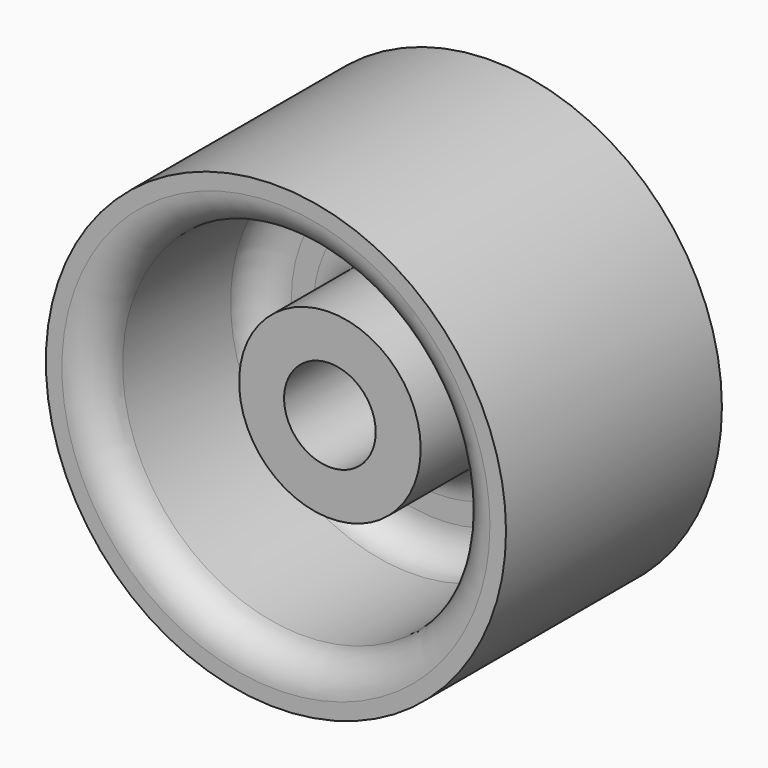
from build123d import *

# Parameters (mm, degrees)
F0_R          = 86.6272823849
F1_DEPTH      = 25.4
F2_R          = 86.6272823849
F2_R_2        = 67.8769245924
F3_DEPTH      = 76.2
F4_R          = 34.1816109176
F4_R_2        = 17.2424518984
F5_DEPTH      = 50.8
F5_DEPTH_BACK = 50.8
F6_R          = 16.8190059926
F7_DEPTH      = 50.8
F8_R          = 12.7
F9_R          = 12.7


with BuildPart() as f1:
    # F0 (on Front) → F1 (new body)
    with BuildSketch(Plane.XZ):
        Circle(F0_R)
    extrude(amount=F1_DEPTH)

    # F2 (on face) → F3 (join)
    with BuildSketch(Plane.XZ.offset(25.4)):
        Circle(F2_R)
        Circle(F2_R_2, mode=Mode.SUBTRACT)
    extrude(amount=F3_DEPTH)

    # F4 (on face) → F5 (join, two sides)
    with BuildSketch(Plane.XZ.offset(25.4)) as f5_sk:
        Circle(F4_R)
        Circle(F4_R_2, mode=Mode.SUBTRACT)
    extrude(amount=F5_DEPTH)
    extrude(f5_sk.sketch, amount=-F5_DEPTH_BACK)

    # F6 (on face) → F7 (cut)
    with BuildSketch(Plane.XZ.offset(25.4)):
        Circle(F6_R)
    extrude(amount=-F7_DEPTH, mode=Mode.SUBTRACT)

    # F8
    f8_edges = [f1.edges().sort_by_distance(p)[0] for p in [
        (-67.876925, -101.6, 0),
    ]]
    fillet(f8_edges, radius=F8_R)

    # F9
    f9_edges = [f1.edges().sort_by_distance(p)[0] for p in [
        (-67.876925, -25.4, 0),
        (-34.181611, -25.4, 0),
    ]]
    fillet(f9_edges, radius=F9_R)


solid = f1.part
